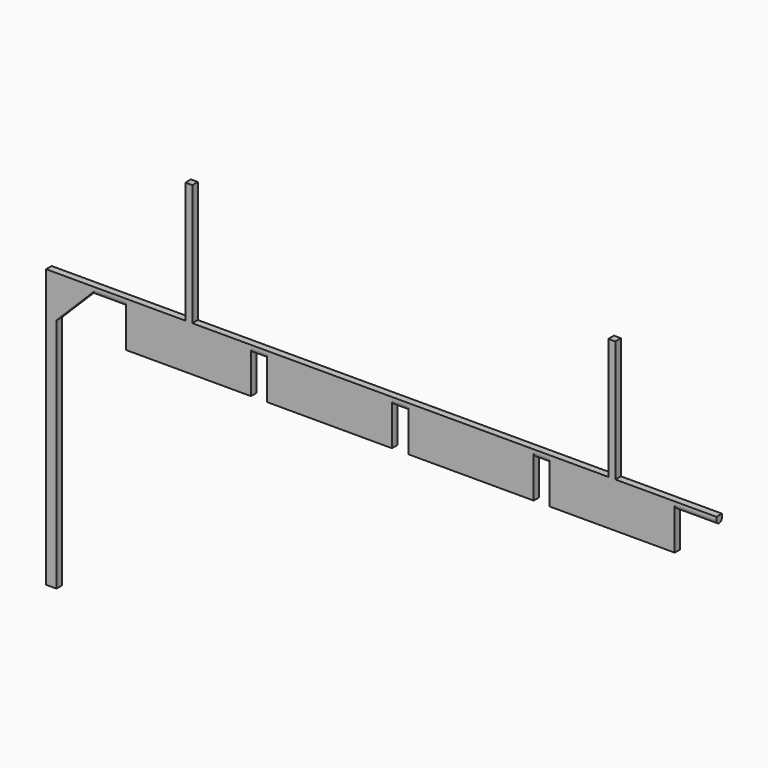
from build123d import *

# Parameters (mm, degrees)
F1_DEPTH = 2
F2_R     = 0.99999
F3_R     = 0.99999


# Not quite as in the source:
# - a fillet or chamfer is up to 0.001 mm smaller than in the source, because OpenCascade refuses the exact size


with BuildPart() as f1:
    # F0 (on Front) → F1 (new body)
    with BuildSketch(Plane.XZ):
        Polygon((59.9, 0), (0, 0), (-59.9, 0), (-59.9, 35), (-61.9, 35), (-61.9, 0), (-79, 0), (-100, 0), (-102, 0), (-102, -80), (-99, -80), (-99, -12), (-89, -2), (-79, -2), (-79, -13), (-43, -13), (-43, -2), (-38.4, -2), (-38.4, -13), (-2.4, -13), (-2.4, -2), (0, -2), (2.4, -2), (2.4, -13), (38.4, -13), (38.4, -2), (43, -2), (43, -13), (79, -13), (79, -2), (91, -2), (91, 0), (79, 0), (61.9, 0), (61.9, 35), (59.9, 35), align=None)
    extrude(amount=F1_DEPTH)

    # F2 (radius 1 in the source; OpenCascade refuses exactly that, so slightly less here)
    f2_edges = [f1.edges().sort_by_distance(p)[0] for p in [
        (-84, -2, -2),
        (-84, 0, -2),
        (85, 0, -2),
        (85, -2, -2),
    ]]
    fillet(f2_edges, radius=F2_R)

    # F3 (radius 1 in the source; OpenCascade refuses exactly that, so slightly less here)
    f3_edges = [f1.edges().sort_by_distance(p)[0] for p in [
        (-40.7, -2, -2),
        (0, -2, -2),
        (40.7, -2, -2),
        (-40.7, 0, -2),
        (0, 0, -2),
        (40.7, 0, -2),
    ]]
    fillet(f3_edges, radius=F3_R)


solid = f1.part
